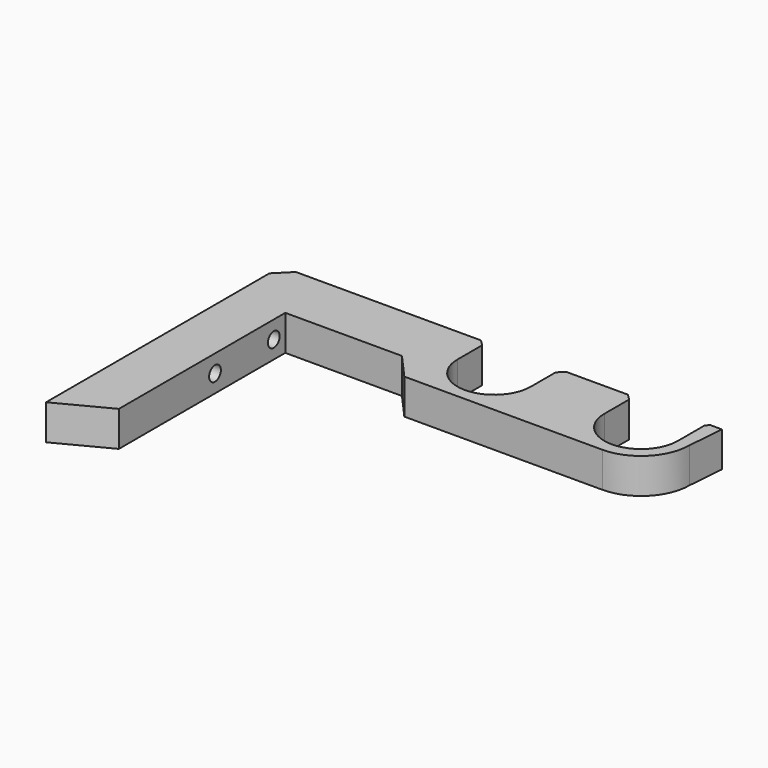
from build123d import *

# Parameters (mm, degrees)
F1_DEPTH = 12
F2_DEPTH = 25
F3_R     = 2.5
F4_DEPTH = 25


# Not quite as in the source:
# - a feature names something its author has since deleted; it is built from what else it names


with BuildPart() as f1:
    # F0 (on Top) → F1 (new body)
    with BuildSketch(Plane.XY):
        with BuildLine():
            Line((5, 0), (0, -5))
            Line((0, -5), (0, -30))
            Line((0, -30), (0, -35))
            Line((0, -35), (0, -60))
            Line((0, -60), (0, -65))
            Line((0, -65), (0, -100))
            Line((0, -100), (17.4887780242, -90.9055213439))
            Line((17.4887780242, -90.9055213439), (17.4887780242, -46.2056212127))
            Line((17.4887780242, -46.2056212127), (17.4887780242, -29))
            Line((17.4887780242, -29), (17.4887780242, -20.1109461486))
            Line((17.4887780242, -20.1109461486), (57.2072267532, -20.1109461486))
            Line((57.2072267532, -20.1109461486), (65.1114210486, -29))
            Line((65.1114210486, -29), (132.5, -29))
            ThreePointArc((132.5, -29), (144.1672618896, -24.1672618896), (149, -12.5))
            Line((149, -12.5), (150, 0))
            Line((150, 0), (145.9653675556, 0))
            Line((145.9653675556, 0), (145, -1.1582256993))
            Line((145, -1.1582256993), (145, -3.3333333333))
            Line((145, -3.3333333333), (145, -12.5))
            ThreePointArc((145, -12.5), (132.5, -25), (120, -12.5))
            Line((120, -12.5), (120, -2))
            Line((120, -2), (118, 0))
            Line((118, 0), (97, 0))
            Line((97, 0), (95, -2))
            Line((95, -2), (95, -12.5))
            ThreePointArc((95, -12.5), (82.5, -25), (70, -12.5))
            Line((70, -12.5), (70, -2))
            Line((70, -2), (68, 0))
            Line((68, 0), (5, 0))
        make_face()
    extrude(amount=F1_DEPTH)

    # F0 (on Top) → F2 (cut)
    with BuildSketch(Plane.XY):
        Polygon((17.4887780242, -46.2056212127), (17.4887780242, -90.9055213439), (27.4864036634, -85.7065764627), (108.4292656183, -38.1771444678), (132.5, -29), (65.1114210486, -29), (57.2072267532, -29), (57.2072267532, -46.2056212127), align=None)
    extrude(amount=-F2_DEPTH, mode=Mode.SUBTRACT)

    # F3 (on face) → F4 (cut)
    with BuildSketch(Plane(origin=(0, 0, 0), x_dir=(0, -1, 0), z_dir=(-1, 0, 0))):
        with Locations((25, 6)):
            Circle(F3_R)
        with Locations((50, 6)):
            Circle(F3_R)
    extrude(amount=-F4_DEPTH, mode=Mode.SUBTRACT)


solid = f1.part
